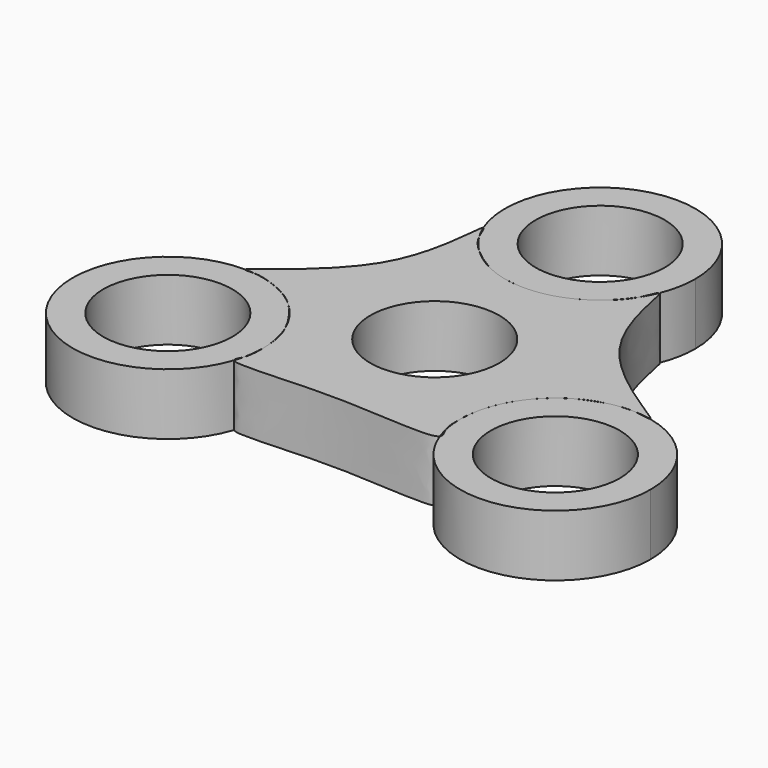
from build123d import *

# Parameters (mm, degrees)
F0_R     = 15.5
F1_DEPTH = 10
F0_R_2   = 10.5
F2_DEPTH = 10
F3_D     = 21


with BuildPart() as f1:
    # F0 (on Top) → F1 (new body)
    with BuildSketch(Plane.XY):
        with BuildLine():
            ThreePointArc((-15.5582190245, -14.3264890886), (-15.5481134615, -14.4614520519), (-15.5391867235, -14.5964981078))
            add(Edge.make_bspline(
                [(-15.8924579792, -18.9743854311), (-15.470540944, -17.8375807671), (-15.4381988559, -16.1449002113), (-15.5391867235, -14.5964981078)],
                knots=[0.8168029759, 0.8168029759, 0.8168029759, 0.8168029759, 0.8443037665, 0.8443037665, 0.8443037665, 0.8443037665], degree=3))
            ThreePointArc((-15.8924579792, -18.9743854311), (-16.0794130092, -19.7148416445), (-16.3026127204, -20.4451905174))
            add(Edge.make_bspline(
                [(17.1873061432, -20.4451905174), (16.3014298673, -21.7117414736), (0.0218349193, -19.3297127556), (-15.5048667998, -21.4166128481), (-16.3026127204, -20.4451905174)],
                knots=[0.6897903941, 0.6897903941, 0.6897903941, 0.6897903941, 0.7456942164, 0.8001402444, 0.8001402444, 0.8001402444, 0.8001402444], degree=3))
            ThreePointArc((17.1873061432, -20.4451905174), (16.8813316533, -19.5064053816), (16.6357506473, -18.5500435834))
            add(Edge.make_bspline(
                [(16.2684202759, -15.5513064952), (16.2423540711, -16.6271780151), (16.2564494045, -17.6188099598), (16.6357506473, -18.5500435834)],
                knots=[0.6474075646, 0.6474075646, 0.6474075646, 0.6474075646, 0.6708457422, 0.6708457422, 0.6708457422, 0.6708457422], degree=3))
            ThreePointArc((16.2684202759, -15.5513064952), (16.3377325298, -13.6635028121), (16.6361801046, -11.7981513762))
            add(Edge.make_bspline(
                [(17.8692555207, -8.3055503859), (17.3272189284, -9.394553247), (16.8932406409, -10.5653192829), (16.6361801046, -11.7981513763)],
                knots=[0.5952695938, 0.5952695938, 0.5952695938, 0.5952695938, 0.6212213126, 0.6212213126, 0.6212213126, 0.6212213126], degree=3))
            ThreePointArc((17.8692555207, -8.3055503859), (18.222794865, -7.6325308147), (18.6089085796, -6.9776555512))
            add(Edge.make_bspline(
                [(19.6971353282, -5.4465283445), (19.3098464213, -5.9223267113), (18.9456042751, -6.4352428588), (18.6089085796, -6.9776555512)],
                knots=[0.5704293982, 0.5704293982, 0.5704293982, 0.5704293982, 0.5843469424, 0.5843469424, 0.5843469424, 0.5843469424], degree=3))
            ThreePointArc((19.6971353282, -5.4465283445), (20.6544483392, -4.3662148965), (21.708105685, -3.3796392304))
            add(Edge.make_bspline(
                [(24.0795047888, -1.7139753765), (23.0341019838, -2.2544156086), (22.383900987, -2.7764853893), (21.708105685, -3.3796392304)],
                knots=[0.5245751869, 0.5245751869, 0.5245751869, 0.5245751869, 0.5475303918, 0.5475303918, 0.5475303918, 0.5475303918], degree=3))
            ThreePointArc((24.0795047888, -1.7139753765), (26.1592440994, -0.7238189892), (28.3627566279, -0.0528064646))
            add(Edge.make_bspline(
                [(29.4819996216, 0.1560571813), (29.1280156413, 0.1057758074), (28.8488211649, 0.0758589623), (28.3627566279, -0.0528064646)],
                knots=[0.4819562631, 0.4819562631, 0.4819562631, 0.4819562631, 0.4956725356, 0.4956725356, 0.4956725356, 0.4956725356], degree=3))
            ThreePointArc((29.4819996216, 0.1560571813), (29.5346038579, 0.1637944926), (29.5872343263, 0.1713513084))
            add(Edge.make_bspline(
                [(32.1982235793, 0.3188527305), (31.0252567727, 0.4279652085), (30.1772464598, 0.25933974), (29.5872343263, 0.1713513084)],
                knots=[0.4588210374, 0.4588210374, 0.4588210374, 0.4588210374, 0.4806275436, 0.4806275436, 0.4806275436, 0.4806275436], degree=3))
            ThreePointArc((32.1982235793, 0.3188527305), (33.6443566585, 0.2104434272), (35.0740285535, -0.0326444841))
            add(Edge.make_bspline(
                [(14.3619581632, 27.8193682397), (15.0243501263, 27.6278227819), (15.5971140402, 10.0587492191), (35.4927930969, 0.4673738297), (35.0878994606, -0.0238765309), (35.0740285535, -0.0326444841)],
                knots=[0.3216986437, 0.3216986437, 0.3216986437, 0.3216986437, 0.375518321, 0.4357800504, 0.4371367656, 0.4371367656, 0.4371367656, 0.4371367656], degree=3))
            ThreePointArc((14.3619581632, 27.8193682397), (13.7777152728, 26.5479361026), (13.0811930675, 25.3343726507))
            add(Edge.make_bspline(
                [(8.418564719, 20.6344400811), (10.3236529663, 21.8410878021), (12.0702297909, 23.4500552065), (13.0811930675, 25.3343726507)],
                knots=[0.2644562413, 0.2644562413, 0.2644562413, 0.2644562413, 0.2991522205, 0.2991522205, 0.2991522205, 0.2991522205], degree=3))
            ThreePointArc((8.418564719, 20.6344400811), (6.5286724505, 19.5909945167), (4.5121342237, 18.8202513607))
            add(Edge.make_bspline(
                [(2.158962907, 18.3000566921), (2.9679292121, 18.4126006012), (3.7517406694, 18.5872633947), (4.5121342237, 18.8202513607)],
                knots=[0.2296025253, 0.2296025253, 0.2296025253, 0.2296025253, 0.2420117038, 0.2420117038, 0.2420117038, 0.2420117038], degree=3))
            ThreePointArc((2.158962907, 18.3000566921), (0.7618708874, 18.1676969397), (-0.6414663653, 18.1622407194))
            add(Edge.make_bspline(
                [(-5.1604492335, 19.0332246604), (-3.7188933237, 18.5035787948), (-2.1741039293, 18.2218682224), (-0.6414663653, 18.1622407194)],
                knots=[0.1930296043, 0.1930296043, 0.1930296043, 0.1930296043, 0.2156331449, 0.2156331449, 0.2156331449, 0.2156331449], degree=3))
            ThreePointArc((-5.1604492335, 19.0332246604), (-8.1422354309, 20.4597992114), (-10.7537265247, 22.4861945685))
            add(Edge.make_bspline(
                [(-13.2797151062, 25.6552660775), (-12.6596986378, 24.3688246089), (-11.8726595212, 23.4698520881), (-10.7537265247, 22.4861945685)],
                knots=[0.1313113839, 0.1313113839, 0.1313113839, 0.1313113839, 0.1584573249, 0.1584573249, 0.1584573249, 0.1584573249], degree=3))
            ThreePointArc((-13.2797151062, 25.6552660775), (-13.8631295105, 26.7161669689), (-14.3619581632, 27.8193682397))
            add(Edge.make_bspline(
                [(-30.7941192418, -0.0528064646), (-30.8697063903, 0.7182307966), (-14.0318115026, 10.3070911944), (-14.9294316383, 27.6791850921), (-14.3619581632, 27.8193682397)],
                knots=[0, 0, 0, 0, 0.0571499927, 0.1103359147, 0.1103359147, 0.1103359147, 0.1103359147], degree=3))
            ThreePointArc((-30.7941192418, -0.0528064646), (-30.0231622661, -0.0827369484), (-29.2546497724, -0.1509941044))
            add(Edge.make_bspline(
                [(-26.3345335257, -0.7732028606), (-27.2700446577, -0.4422069705), (-28.2256027607, -0.1601777804), (-29.2546497724, -0.1509941044)],
                knots=[0.9599518266, 0.9599518266, 0.9599518266, 0.9599518266, 0.9832519631, 0.9832519631, 0.9832519631, 0.9832519631], degree=3))
            ThreePointArc((-26.3345335257, -0.7732028606), (-24.9283553379, -1.294145701), (-23.5790984648, -1.9485342928))
            add(Edge.make_bspline(
                [(-20.5137407688, -4.1458787741), (-21.575808525, -3.0915788756), (-22.567664452, -2.4681673894), (-23.5790984648, -1.9485342928)],
                knots=[0.910425059, 0.910425059, 0.910425059, 0.910425059, 0.9366128391, 0.9366128391, 0.9366128391, 0.9366128391], degree=3))
            ThreePointArc((-20.5137407688, -4.1458787741), (-18.3031787998, -6.6747622476), (-16.6893013472, -9.6204770011))
            add(Edge.make_bspline(
                [(-15.5582190245, -14.3264890886), (-15.6830341709, -12.6769515602), (-15.9455659909, -11.2429506099), (-16.6893013472, -9.6204770011)],
                knots=[0.8459118787, 0.8459118787, 0.8459118787, 0.8459118787, 0.8755780604, 0.8755780604, 0.8755780604, 0.8755780604], degree=3))
        make_face()
        Circle(F0_R, mode=Mode.SUBTRACT)
    extrude(amount=F1_DEPTH)

    # F0 (on Top) → F2, piece 4 (join)
    with BuildSketch(Plane.XY):
        Circle(F0_R)
        Circle(F0_R_2, mode=Mode.SUBTRACT)
    extrude(amount=F2_DEPTH)


with BuildPart() as f2:
    # F0 (on Top) → F2 (new body)
    with BuildSketch(Plane.XY):
        with BuildLine():
            ThreePointArc((-15.8924579792, -18.9743854311), (-15.6057244357, -17.2735096249), (-15.5097504153, -15.5513064952))
            ThreePointArc((-15.5097504153, -15.5513064952), (-15.5171112402, -15.0736754783), (-15.5391867235, -14.5964981078))
            add(Edge.make_bspline(
                [(-15.5391867235, -14.5964981078), (-15.5450920018, -14.5059550998), (-15.5514531805, -14.415905429), (-15.5582190245, -14.3264890886)],
                knots=[0.8443037665, 0.8443037665, 0.8443037665, 0.8443037665, 0.8459118787, 0.8459118787, 0.8459118787, 0.8459118787], degree=3))
            ThreePointArc((-15.5582190245, -14.3264890886), (-15.9389394699, -11.9290616875), (-16.6893013472, -9.6204770011))
            add(Edge.make_bspline(
                [(-16.6893013472, -9.6204770011), (-17.5629205098, -7.7146592618), (-19.1004910215, -5.5487921537), (-20.5137407688, -4.1458787741)],
                knots=[0.8755780604, 0.8755780604, 0.8755780604, 0.8755780604, 0.910425059, 0.910425059, 0.910425059, 0.910425059], degree=3))
            ThreePointArc((-20.5137407688, -4.1458787741), (-21.9793362666, -2.9536233628), (-23.5790984648, -1.9485342928))
            add(Edge.make_bspline(
                [(-23.5790984648, -1.9485342928), (-24.4805053703, -1.4854285877), (-25.3974625079, -1.1047506583), (-26.3345335257, -0.7732028606)],
                knots=[0.9366128391, 0.9366128391, 0.9366128391, 0.9366128391, 0.9599518266, 0.9599518266, 0.9599518266, 0.9599518266], degree=3))
            ThreePointArc((-26.3345335257, -0.7732028606), (-27.7795752147, -0.3916241709), (-29.2546497724, -0.1509941044))
            add(Edge.make_bspline(
                [(-29.2546497724, -0.1509941044), (-29.994324293, -0.144392918), (-30.7719681217, -0.2787620577), (-30.7941192418, -0.0528064646)],
                knots=[0.9832519631, 0.9832519631, 0.9832519631, 0.9832519631, 1, 1, 1, 1], degree=3))
            ThreePointArc((-30.7941192418, -0.0528064646), (-43.644408682, -24.529914989), (-16.3026127204, -20.4451905174))
            add(Edge.make_bspline(
                [(-16.3026127204, -20.4451905174), (-16.546755894, -20.1478951949), (-16.148097549, -19.6631754796), (-15.8924579792, -18.9743854311)],
                knots=[0.8001402444, 0.8001402444, 0.8001402444, 0.8001402444, 0.8168029759, 0.8168029759, 0.8168029759, 0.8168029759], degree=3))
        make_face()
        with Locations((-31.0097504153, -15.5513064952)):
            Circle(F0_R_2, mode=Mode.SUBTRACT)
        with Locations((-31.0097504153, -15.5513064952)):
            Circle(F0_R_2)
        with BuildLine():
            add(Edge.make_bspline(
                [(-15.5391867235, -14.5964981078), (-15.5450920018, -14.5059550998), (-15.5514531805, -14.415905429), (-15.5582190245, -14.3264890886)],
                knots=[0.8443037665, 0.8443037665, 0.8443037665, 0.8443037665, 0.8459118787, 0.8459118787, 0.8459118787, 0.8459118787], degree=3))
            ThreePointArc((-15.5391867235, -14.5964981078), (-15.5481134615, -14.4614520519), (-15.5582190245, -14.3264890886))
        make_face()
    extrude(amount=F2_DEPTH)

    # F3 (through all)
    with Locations(Plane(origin=(0, 0, 0), x_dir=(1, 0, 0), z_dir=(0, 0, -1))):
        with Locations((0, -33.6489615118), (0, 0), (31.7638530981, 15.1750596962), (-31.0097504153, 15.5513064952)):
            Hole(F3_D / 2)


with BuildPart() as f2b:
    # F0 (on Top) → F2, piece 2 (new body)
    with BuildSketch(Plane.XY):
        with BuildLine():
            add(Edge.make_bspline(
                [(16.6357506473, -18.5500435834), (16.9423329315, -19.3027427556), (17.4875113353, -20.0159825305), (17.1873061432, -20.4451905174)],
                knots=[0.6708457422, 0.6708457422, 0.6708457422, 0.6708457422, 0.6897903941, 0.6897903941, 0.6897903941, 0.6897903941], degree=3))
            ThreePointArc((17.1873061432, -20.4451905174), (34.4390654448, -30.4424510549), (47.2638530981, -15.1750596962))
            ThreePointArc((47.2638530981, -15.1750596962), (43.8377447565, -5.4554331488), (35.0740285535, -0.0326444841))
            add(Edge.make_bspline(
                [(35.0740285535, -0.0326444841), (34.8523309414, -0.1727819868), (33.3646154234, 0.2103518728), (32.1982235793, 0.3188527305)],
                knots=[0.4371367656, 0.4371367656, 0.4371367656, 0.4371367656, 0.4588210374, 0.4588210374, 0.4588210374, 0.4588210374], degree=3))
            ThreePointArc((32.1982235793, 0.3188527305), (30.8896126026, 0.3002659403), (29.5872343263, 0.1713513084))
            add(Edge.make_bspline(
                [(29.5872343263, 0.1713513084), (29.5512835598, 0.1659899754), (29.5162906732, 0.1609280266), (29.4819996216, 0.1560571813)],
                knots=[0.4806275436, 0.4806275436, 0.4806275436, 0.4806275436, 0.4819562631, 0.4819562631, 0.4819562631, 0.4819562631], degree=3))
            ThreePointArc((29.4819996216, 0.1560571813), (28.9204596976, 0.0619056831), (28.3627566279, -0.0528064646))
            add(Edge.make_bspline(
                [(28.3627566279, -0.0528064646), (27.3385312948, -0.3239276422), (25.3957602034, -1.0335128999), (24.0795047888, -1.7139753765)],
                knots=[0.4956725356, 0.4956725356, 0.4956725356, 0.4956725356, 0.5245751869, 0.5245751869, 0.5245751869, 0.5245751869], degree=3))
            ThreePointArc((24.0795047888, -1.7139753765), (22.8547926494, -2.4912652355), (21.708105685, -3.3796392304))
            add(Edge.make_bspline(
                [(21.708105685, -3.3796392304), (21.0339648504, -3.9813164434), (20.334354876, -4.6636811862), (19.6971353282, -5.4465283445)],
                knots=[0.5475303918, 0.5475303918, 0.5475303918, 0.5475303918, 0.5704293982, 0.5704293982, 0.5704293982, 0.5704293982], degree=3))
            ThreePointArc((19.6971353282, -5.4465283445), (19.1298058535, -6.1955914368), (18.6089085796, -6.9776555512))
            add(Edge.make_bspline(
                [(18.6089085796, -6.9776555512), (18.3446658579, -7.4033473795), (18.0973898052, -7.8472069972), (17.8692555207, -8.3055503859)],
                knots=[0.5843469424, 0.5843469424, 0.5843469424, 0.5843469424, 0.5952695938, 0.5952695938, 0.5952695938, 0.5952695938], degree=3))
            ThreePointArc((17.8692555207, -8.3055503859), (17.1480187842, -10.0148865103), (16.6361801046, -11.7981513762))
            add(Edge.make_bspline(
                [(16.6361801046, -11.7981513763), (16.376796438, -13.0421249287), (16.2975426854, -14.3492914254), (16.2684202759, -15.5513064952)],
                knots=[0.6212213126, 0.6212213126, 0.6212213126, 0.6212213126, 0.6474075646, 0.6474075646, 0.6474075646, 0.6474075646], degree=3))
            ThreePointArc((16.2684202759, -15.5513064952), (16.3788495497, -17.0596460741), (16.6357506473, -18.5500435834))
        make_face()
        with Locations((31.7638530981, -15.1750596962)):
            Circle(F0_R_2, mode=Mode.SUBTRACT)
    extrude(amount=F2_DEPTH)


with BuildPart() as f2c:
    # F0 (on Top) → F2, piece 3 (new body)
    with BuildSketch(Plane.XY):
        with BuildLine():
            ThreePointArc((15.5, 33.6489615118), (-2.9698188893, 48.8617908267), (-14.3619581632, 27.8193682397))
            add(Edge.make_bspline(
                [(-14.3619581632, 27.8193682397), (-14.1381579176, 27.8746536835), (-13.7587972767, 26.64928995), (-13.2797151062, 25.6552660775)],
                knots=[0.1103359147, 0.1103359147, 0.1103359147, 0.1103359147, 0.1313113839, 0.1313113839, 0.1313113839, 0.1313113839], degree=3))
            ThreePointArc((-13.2797151062, 25.6552660775), (-12.1207397759, 23.9878193803), (-10.7537265247, 22.4861945685))
            add(Edge.make_bspline(
                [(-10.7537265247, 22.4861945685), (-9.3286860679, 21.2334370168), (-7.3653194691, 19.8433218594), (-5.1604492335, 19.0332246604)],
                knots=[0.1584573249, 0.1584573249, 0.1584573249, 0.1584573249, 0.1930296043, 0.1930296043, 0.1930296043, 0.1930296043], degree=3))
            ThreePointArc((-5.1604492335, 19.0332246604), (-2.9334637223, 18.4290800869), (-0.6414663653, 18.1622407194))
            add(Edge.make_bspline(
                [(-0.6414663653, 18.1622407194), (0.305730255, 18.1253898875), (1.2482855388, 18.1733626749), (2.158962907, 18.3000566921)],
                knots=[0.2156331449, 0.2156331449, 0.2156331449, 0.2156331449, 0.2296025253, 0.2296025253, 0.2296025253, 0.2296025253], degree=3))
            ThreePointArc((2.158962907, 18.3000566921), (3.3456740509, 18.5143500155), (4.5121342237, 18.8202513607))
            add(Edge.make_bspline(
                [(4.5121342237, 18.8202513607), (5.8874614871, 19.2416577491), (7.1861791406, 19.85386981), (8.418564719, 20.6344400811)],
                knots=[0.2420117038, 0.2420117038, 0.2420117038, 0.2420117038, 0.2644562413, 0.2644562413, 0.2644562413, 0.2644562413], degree=3))
            ThreePointArc((8.418564719, 20.6344400811), (11.0037374451, 22.7325627357), (13.0811930675, 25.3343726507))
            add(Edge.make_bspline(
                [(13.0811930675, 25.3343726507), (13.7381454388, 26.5588551238), (14.0844654273, 27.8996114735), (14.3619581632, 27.8193682397)],
                knots=[0.2991522205, 0.2991522205, 0.2991522205, 0.2991522205, 0.3216986437, 0.3216986437, 0.3216986437, 0.3216986437], degree=3))
            ThreePointArc((14.3619581632, 27.8193682397), (15.2128293149, 30.6791426226), (15.5, 33.6489615118))
        make_face()
        with Locations((0, 33.6489615118)):
            Circle(F0_R_2, mode=Mode.SUBTRACT)
    extrude(amount=F2_DEPTH)


solid = Compound([f1.part, f2.part, f2b.part, f2c.part])
